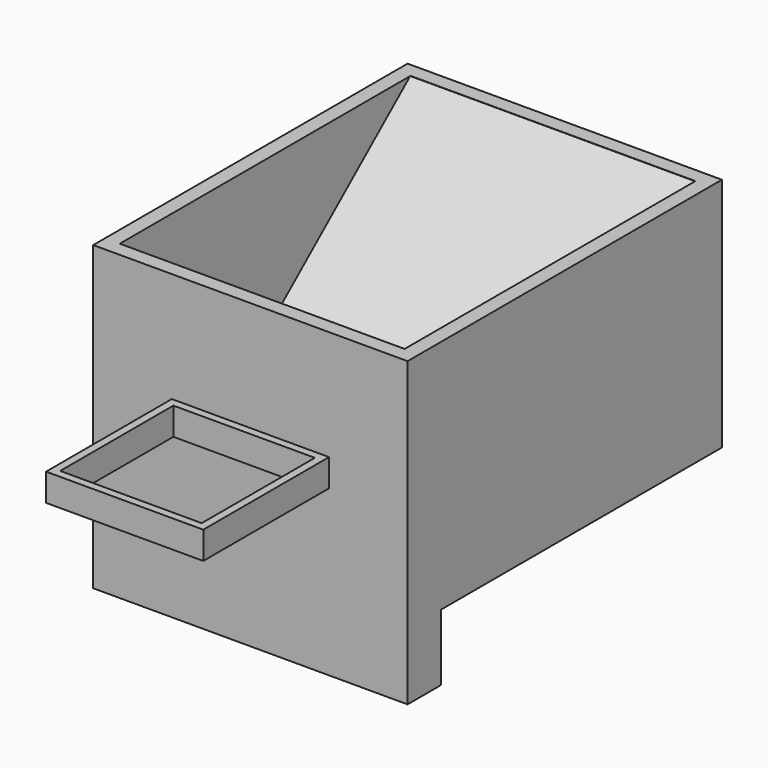
from build123d import *

# Parameters (mm, degrees)
F0_W      = 101.6
F0_H      = 76.2
F1_DEPTH  = 127
F2_T      = -4.7625
F4_DEPTH  = 101.6
F5_W      = 50.8
F5_H      = 8.89
F6_DEPTH  = 50.8
F7_W      = 45.72
F7_H      = 45.72
F8_DEPTH  = 25.4
F11_W     = 13.5890031233
F11_H     = 21.4630011469
F12_DEPTH = 101.6


# Not quite as in the source:
# - the program builds the solid bodies; features that only make, move or delete a surface that nothing else refers to are left out


with BuildPart() as f1:
    # F0 (on Front) → F1 (new body)
    with BuildSketch(Plane.XZ):
        with Locations((50.8, 38.1)):
            Rectangle(F0_W, F0_H)
    extrude(amount=-F1_DEPTH)

    # F2
    f2_openings = [f1.faces().sort_by_distance(p)[0] for p in [
        (50.8, 63.5, 76.2),
    ]]
    offset(amount=F2_T, openings=f2_openings)

    # F3 (on face) → F4 (join)
    with BuildSketch(Plane.YZ.offset(101.6)):
        Polygon((122.1133470535, 0), (122.1133470535, 76.2), (31.75, 0), align=None)
    extrude(amount=-F4_DEPTH)

    # F5 (on face) → F6 (join)
    with BuildSketch(Plane.XZ):
        with Locations((50.8, 36.195)):
            Rectangle(F5_W, F5_H)
    extrude(amount=F6_DEPTH)

    # F7 (on face) → F8 (cut)
    with BuildSketch(Plane.XY.offset(40.64)):
        with Locations((50.8, -25.4)):
            Rectangle(F7_W, F7_H)
    extrude(amount=-F8_DEPTH, mode=Mode.SUBTRACT)

    # F11 (on Right) → F12 (join)
    with BuildSketch(Plane.YZ):
        with Locations((6.7945015617, -10.7315005735)):
            Rectangle(F11_W, F11_H)
    extrude(amount=F12_DEPTH)


solid = f1.part
